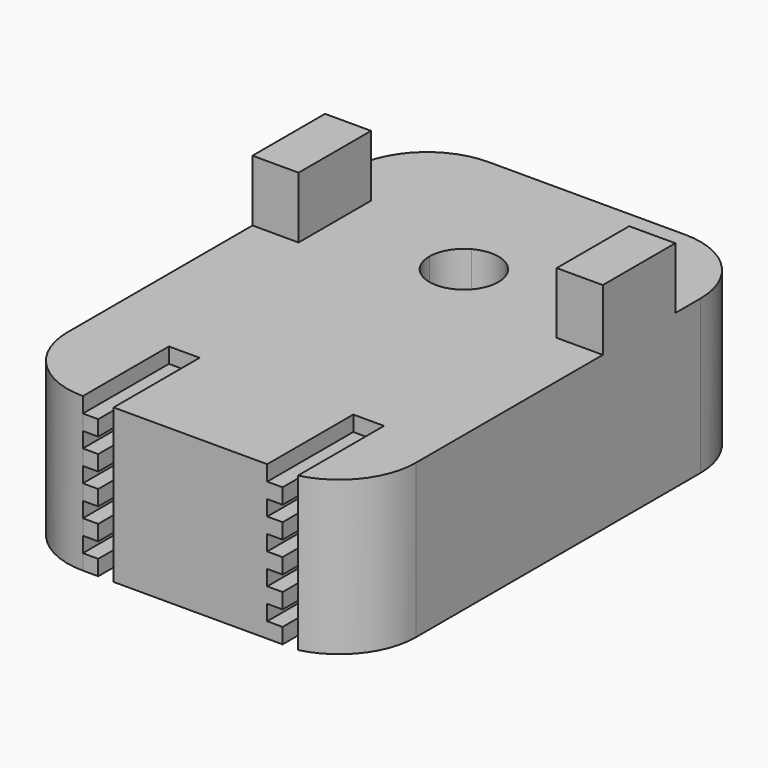
from build123d import *

# Parameters (mm, degrees)
F0_W        = 18.5
F0_H        = 13
F0_W_2      = 4.3
F0_W_3      = 3
F0_H_2      = 2.95
F1_DEPTH    = 10
F3_DEPTH    = 7
F4_T1_DEPTH = 35
F4_T3_DEPTH = 34.269322199
F0_H_3      = 5.9
F5_DEPTH    = 14
F6_R        = 5.5
F7_DEPTH    = 4
F8_SIZE     = 2


# Not quite as in the source:
# - a fillet or chamfer that OpenCascade refuses, or shapes differently, is made with other operations: its cross-section is extruded or revolved along the edge and cut away or added


with BuildPart() as f1:
    # F0 (on Top) → F1 (new body)
    with BuildSketch(Plane.XY):
        with Locations((5.190736489, 6.5)):
            Rectangle(F0_W, F0_H)
        with Locations((16.590736489, 6.5)):
            Rectangle(F0_W_2, F0_H)
        Polygon((14.440736489, 20.05), (14.440736489, 13), (18.740736489, 13), (18.740736489, 20.05), (15.740736489, 20.05), (15.740736489, 25.95), (18.740736489, 25.95), (18.740736489, 33), (14.440736489, 33), (14.440736489, 25.95), (14.440736489, 23), align=None)
        with BuildLine():
            Line((-4.059263511, 20.05), (-4.059263511, 13))
            Line((-4.059263511, 13), (14.440736489, 13))
            Line((14.440736489, 13), (14.440736489, 20.05))
            Line((14.440736489, 20.05), (11.440736489, 20.05))
            Line((11.440736489, 20.05), (11.440736489, 23))
            Line((11.440736489, 23), (9.590736489, 23))
            ThreePointArc((9.590736489, 23), (8.4904647177, 21.0659304563), (6.265736489, 21.0234183548))
            ThreePointArc((6.265736489, 21.0234183548), (4.0410082602, 21.0659304563), (2.940736489, 23))
            Line((2.940736489, 23), (-1.059263511, 23))
            Line((-1.059263511, 23), (-1.059263511, 20.05))
            Line((-1.059263511, 20.05), (-4.059263511, 20.05))
        make_face()
        with Locations((12.940736489, 21.525)):
            Rectangle(F0_W_3, F0_H_2)
        with Locations((12.940736489, 24.475)):
            Rectangle(F0_W_3, F0_H_2)
        with BuildLine():
            Line((-4.059263511, 33), (-4.059263511, 25.95))
            Line((-4.059263511, 25.95), (-1.059263511, 25.95))
            Line((-1.059263511, 25.95), (-1.059263511, 23))
            Line((-1.059263511, 23), (2.940736489, 23))
            ThreePointArc((2.940736489, 23), (4.0410082602, 24.9340695437), (6.265736489, 24.9765816452))
            ThreePointArc((6.265736489, 24.9765816452), (8.4904647177, 24.9340695437), (9.590736489, 23))
            Line((9.590736489, 23), (11.440736489, 23))
            Line((11.440736489, 23), (11.440736489, 25.95))
            Line((11.440736489, 25.95), (14.440736489, 25.95))
            Line((14.440736489, 25.95), (14.440736489, 33))
            Line((14.440736489, 33), (-4.059263511, 33))
        make_face()
        with BuildLine():
            Line((5.090736489, 23), (2.940736489, 23))
            ThreePointArc((2.940736489, 23), (4.0410082602, 21.0659304563), (6.265736489, 21.0234183548))
            ThreePointArc((6.265736489, 21.0234183548), (5.4066669452, 21.8502717712), (5.090736489, 23))
        make_face()
        with BuildLine():
            ThreePointArc((6.265736489, 24.9765816452), (4.0410082602, 24.9340695437), (2.940736489, 23))
            Line((2.940736489, 23), (5.090736489, 23))
            ThreePointArc((5.090736489, 23), (5.4066669452, 24.1497282288), (6.265736489, 24.9765816452))
        make_face()
    extrude(amount=F1_DEPTH)

    # F2 (on face) → F3 (cut)
    with BuildSketch(Plane.XZ):
        Polygon((2.940736489, 10), (0.940736489, 10), (0.940736489, 9), (1.940736489, 9), (1.940736489, 8), (0.940736489, 8), (0.940736489, 7), (1.940736489, 7), (1.940736489, 6), (0.940736489, 6), (0.940736489, 5), (1.940736489, 5), (1.940736489, 4), (0.940736489, 4), (0.940736489, 3), (1.940736489, 3), (1.940736489, 2), (0.940736489, 2), (0.940736489, 1), (1.940736489, 1), (1.940736489, 0), (2.940736489, 0), align=None)
        Polygon((14.940736489, 10), (12.940736489, 10), (12.940736489, 9), (13.940736489, 9), (13.940736489, 8), (12.940736489, 8), (12.940736489, 7), (13.940736489, 7), (13.940736489, 6), (12.940736489, 6), (12.940736489, 5), (13.940736489, 5), (13.940736489, 4), (12.940736489, 4), (12.940736489, 3), (13.940736489, 3), (13.940736489, 2), (12.940736489, 2), (12.940736489, 1), (13.940736489, 1), (13.940736489, 0), (14.940736489, 0), align=None)
    extrude(amount=-F3_DEPTH, mode=Mode.SUBTRACT)

    # F4: fillet of radius 5 on 4 edges, made by hand

    # F4_s2 → F4_t1 (cut)
    with BuildSketch(Plane.XY.offset(-12.5)):
        with BuildLine():
            ThreePointArc((-4.059263511, 28), (-2.594797417, 31.5355339059), (0.940736489, 33))
            Line((0.940736489, 33), (-4.059263511, 33))
            Line((-4.059263511, 33), (-4.059263511, 28))
        make_face()
        with BuildLine():
            ThreePointArc((0.940736489, 0), (-2.594797417, 1.4644660941), (-4.059263511, 5))
            Line((-4.059263511, 5), (-4.059263511, 0))
            Line((-4.059263511, 0), (0.940736489, 0))
        make_face()
        with BuildLine():
            ThreePointArc((13.740736489, 33), (17.2762703949, 31.5355339059), (18.740736489, 28))
            Line((18.740736489, 28), (18.740736489, 33))
            Line((18.740736489, 33), (13.740736489, 33))
        make_face()
    extrude(amount=F4_T1_DEPTH, mode=Mode.SUBTRACT)

    # F4_s4 → F4_t3 (cut)
    with BuildSketch(Plane.XY.offset(-12.1346610995)):
        with BuildLine():
            ThreePointArc((18.740736489, 4.8538644398), (17.677740426, 1.7716574383), (14.940736489, 0))
            Line((14.940736489, 0), (18.740736489, 0))
            Line((18.740736489, 0), (18.740736489, 4.8538644398))
        make_face()
    extrude(amount=F4_T3_DEPTH, mode=Mode.SUBTRACT)

    # F0 (on Top) → F5 (join)
    with BuildSketch(Plane.XY):
        with Locations((-2.559263511, 24.475)):
            Rectangle(F0_W_3, F0_H_2)
        with Locations((-2.559263511, 21.525)):
            Rectangle(F0_W_3, F0_H_2)
        with Locations((17.240736489, 23)):
            Rectangle(F0_W_3, F0_H_3)
    extrude(amount=F5_DEPTH)

    # F6 (on face) → F7 (cut)
    with BuildSketch(Plane(origin=(0, 0, 0), x_dir=(1, 0, 0), z_dir=(0, 0, -1))):
        with Locations((7.340736489, -23)):
            Circle(F6_R)
    extrude(amount=-F7_DEPTH, mode=Mode.SUBTRACT)

    # F8
    f8_edges = [f1.edges().sort_by_distance(p)[0] for p in [
        (1.840736, 23, 4),
    ]]
    chamfer(f8_edges, length=F8_SIZE)


solid = f1.part
